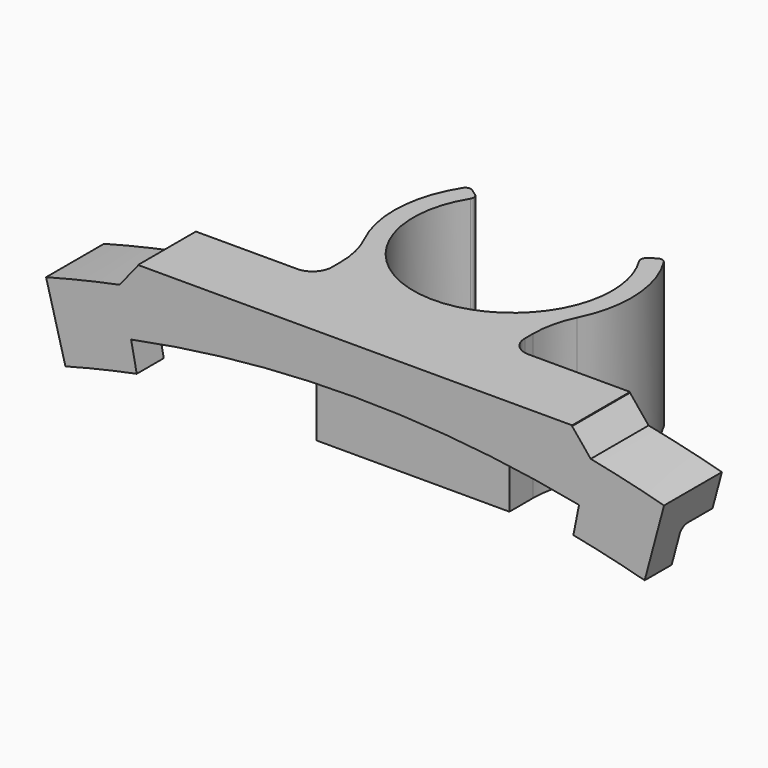
from build123d import *

# Parameters (mm, degrees)
F1_DEPTH       = 9.525
F2_DEPTH       = 9.525
F3_T1_DEPTH    = 19.05
F3_T3_DEPTH    = 9.525
F3_T5_DEPTH    = 9.525
F4_R           = 0.762
F6_W           = 9.525
F6_H           = 3.81
F6_W_2         = 4.445
F7_ANGLE_BACK  = 15
F7_ANGLE       = 30
F8_R           = 1.016
F9_DEPTH       = 28.575
F10_R          = 2.54
F11_T1_DEPTH   = 9.525
F12_ANGLE_BACK = 11.25
F12_ANGLE      = 22.5


# Not quite as in the source:
# - a fillet or chamfer that OpenCascade refuses, or shapes differently, is made with other operations: its cross-section is extruded or revolved along the edge and cut away or added


with BuildPart() as f1:
    # F0 (on Top) → F1 (new body, symmetric)
    with BuildSketch(Plane.XY):
        with BuildLine():
            ThreePointArc((12.7, -9.0953637091), (14.8728333044, -4.7764495705), (15.621, 0))
            ThreePointArc((15.621, 0), (14.8980124876, 4.6973252941), (12.7959740838, 8.9598375122))
            Line((12.7959740838, 8.9598375122), (10.7153278913, 7.5029533639))
            ThreePointArc((10.7153278913, 7.5029533639), (12.4755714327, 3.9335325633), (13.081, 0))
            ThreePointArc((13.081, 0), (-3.9335325633, -12.4755714327), (-10.7153278913, 7.5029533639))
            Line((-10.7153278913, 7.5029533639), (-12.7959740838, 8.9598375122))
            ThreePointArc((-12.7959740838, 8.9598375122), (-15.6207793149, -0.0830336901), (-12.7, -9.0953637091))
            ThreePointArc((-12.7, -9.0953637091), (0, -15.621), (12.7, -9.0953637091))
        make_face()
    extrude(amount=F1_DEPTH, both=True)

    # F0 (on Top) → F2 (join, symmetric)
    with BuildSketch(Plane.XY):
        with BuildLine():
            Line((12.7, -16.4338), (12.7, -9.0953637091))
            ThreePointArc((12.7, -9.0953637091), (0, -15.621), (-12.7, -9.0953637091))
            Line((-12.7, -9.0953637091), (-12.7, -16.4338))
            Line((-12.7, -16.4338), (12.7, -16.4338))
        make_face()
    extrude(amount=F2_DEPTH, both=True)

    # F3: fillet of radius 12.7 on 3 edges, made by hand

    # F3_s2 → F3_t1 (join)
    with BuildSketch(Plane.XY.offset(-9.525)):
        with BuildLine():
            ThreePointArc((-14.0098654709, -6.9093639714), (-13.0318006864, -9.6427001587), (-12.7, -12.5267330538))
            Line((-12.7, -12.5267330538), (-12.7, -9.0953637091))
            ThreePointArc((-12.7, -9.0953637091), (-13.3995849593, -8.0291197475), (-14.0098654709, -6.9093639714))
        make_face()
    extrude(amount=F3_T1_DEPTH)

    # F3_s4 → F3_t3 (join)
    with BuildSketch(Plane.XY):
        with BuildLine():
            ThreePointArc((14.0098654709, -6.9093639714), (13.0318006864, -9.6427001587), (12.7, -12.5267330538))
            Line((12.7, -12.5267330538), (12.7, -9.0953637091))
            ThreePointArc((12.7, -9.0953637091), (13.3995849593, -8.0291197475), (14.0098654709, -6.9093639714))
        make_face()
    extrude(amount=F3_T3_DEPTH)

    # F3_s6 → F3_t5 (join)
    with BuildSketch(Plane.XY.offset(-9.525)):
        with BuildLine():
            ThreePointArc((12.7, -12.5267330538), (13.0318006864, -9.6427001587), (14.0098654709, -6.9093639714))
            ThreePointArc((14.0098654709, -6.9093639714), (13.3995849593, -8.0291197475), (12.7, -9.0953637091))
            Line((12.7, -9.0953637091), (12.7, -12.5267330538))
        make_face()
    extrude(amount=F3_T5_DEPTH)

    # F4
    f4_edges = [f1.edges().sort_by_distance(p)[0] for p in [
        (-12.795974, 8.959838, 0),
        (-10.715328, 7.502953, -4.7625),
        (-10.715328, 7.502953, 4.7625),
        (12.795974, 8.959838, 4.7625),
        (12.795974, 8.959838, -4.7625),
        (10.715328, 7.502953, 4.7625),
        (10.715328, 7.502953, -4.7625),
    ]]
    fillet(f4_edges, radius=F4_R)

    # F6 (on Right) → F7 (revolve)
    with BuildSketch(Plane.YZ, mode=Mode.PRIVATE) as f7_sk:
        with Locations((-21.1963, 7.62)):
            Rectangle(F6_W, F6_H)
        Polygon((-16.4338, 4.7625), (-16.4338, 5.715), (-25.9588, 5.715), (-25.9588, 3.4925), (-21.5138, 3.4925), (-21.5138, 4.7625), align=None)
        with Locations((-23.7363, 1.5875)):
            Rectangle(F6_W_2, F6_H)
    revolve(f7_sk.sketch.rotate(Axis((0, -16.4338, -147.6375), (0, -1, 0)), -F7_ANGLE_BACK), axis=Axis((0, -16.4338, -147.6375), (0, -1, 0)), revolution_arc=F7_ANGLE)

    # F8
    f8_edges = [f1.edges().sort_by_distance(p)[0] for p in [
        (0, -21.5138, 4.7625),
    ]]
    fillet(f8_edges, radius=F8_R)

    # F6 (on Right) → F9 (join, symmetric)
    with BuildSketch(Plane.YZ):
        with Locations((-21.1963, 7.62)):
            Rectangle(F6_W, F6_H)
        Polygon((-16.4338, 4.7625), (-16.4338, 5.715), (-25.9588, 5.715), (-25.9588, 3.4925), (-21.5138, 3.4925), (-21.5138, 4.7625), align=None)
        with Locations((-23.7363, 1.5875)):
            Rectangle(F6_W_2, F6_H)
    extrude(amount=F9_DEPTH, both=True)

    # F10
    f10_edges = [f1.edges().sort_by_distance(p)[0] for p in [
        (-12.7, -16.4338, 6.878706),
        (12.7, -16.4338, 6.878706),
    ]]
    fillet(f10_edges, radius=F10_R)

    # F11: chamfer of 2.54 on 2 edges, made by hand

    # F11_s2 → F11_t1 (join)
    with BuildSketch(Plane.XZ.offset(16.4338)):
        with BuildLine():
            Line((-31.089435357, 6.3536630782), (-28.5106384895, 9.503518522))
            Line((-28.5106384895, 9.503518522), (-28.4598384895, 9.503518522))
            ThreePointArc((-28.4598384895, 9.503518522), (-28.5242, 8.2044800333), (-28.5242, 6.9054415446))
            Line((-28.5242, 6.9054415446), (-28.5657636364, 6.8554882705))
            ThreePointArc((-28.5657636364, 6.8554882705), (-29.8296810134, 6.6164348202), (-31.0794070503, 6.3038627463))
            Line((-31.0794070503, 6.3038627463), (-31.089435357, 6.3536630782))
        make_face()
        with BuildLine():
            Line((31.089435357, 6.3536630782), (28.5106384895, 9.503518522))
            Line((28.5106384895, 9.503518522), (28.4598384895, 9.503518522))
            ThreePointArc((28.4598384895, 9.503518522), (28.5242, 8.2044800333), (28.5242, 6.9054415446))
            Line((28.5242, 6.9054415446), (28.5657636364, 6.8554882705))
            ThreePointArc((28.5657636364, 6.8554882705), (29.8296810134, 6.6164348202), (31.0794070503, 6.3038627463))
            Line((31.0794070503, 6.3038627463), (31.089435357, 6.3536630782))
        make_face()
    extrude(amount=F11_T1_DEPTH)

    # F6 (on Right) → F12 (revolve, cut)
    with BuildSketch(Plane.YZ, mode=Mode.PRIVATE) as f12_sk:
        with Locations((-23.7363, 1.5875)):
            Rectangle(F6_W_2, F6_H)
    revolve(f12_sk.sketch.rotate(Axis((0, -25.9588, -147.6375), (0, 1, 0)), -F12_ANGLE_BACK), axis=Axis((0, -25.9588, -147.6375), (0, 1, 0)), revolution_arc=F12_ANGLE, mode=Mode.SUBTRACT)


solid = f1.part
